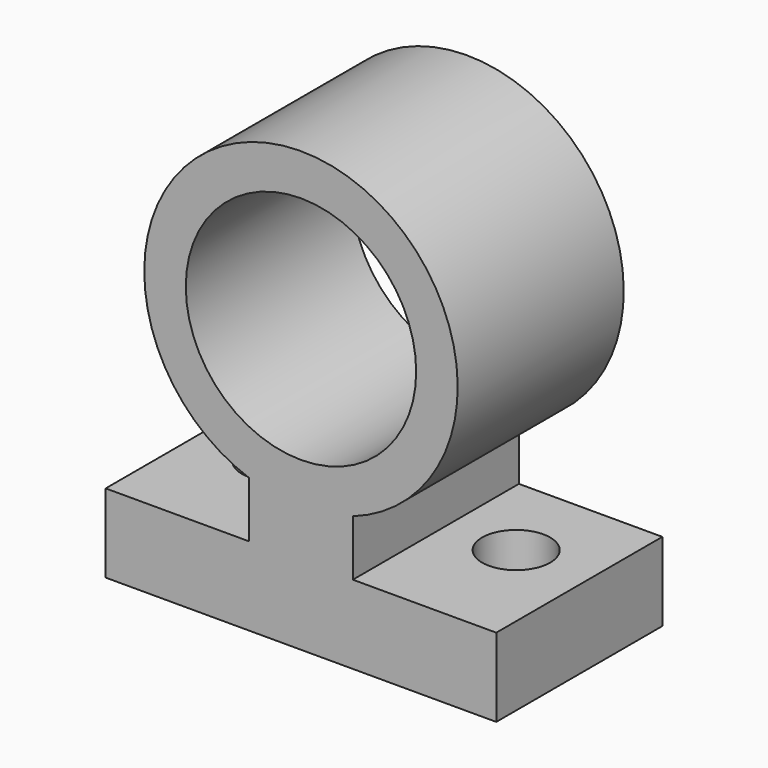
from build123d import *

# Parameters (mm, degrees)
F1_DEPTH = 25.4
F2_R     = 4.1683581246
F3_DEPTH = 10.668


# Not quite as in the source:
# - a feature names something its author has since deleted; it is built from what else it names


with BuildPart() as f1:
    # F0 (on Front) → F1 (new body)
    with BuildSketch(Plane.XZ):
        with BuildLine():
            ThreePointArc((6.35, -18.0951603751), (11.0901618338, 15.6449876798), (-19.177, 0))
            ThreePointArc((-19.177, 0), (-15.6449876798, -11.0901618338), (-6.35, -18.0951603751))
            Line((-6.35, -18.0951603751), (-6.35, -24.9301567674))
            Line((-6.35, -24.9301567674), (-23.899981752, -24.9301567674))
            Line((-23.899981752, -24.9301567674), (-23.899981752, -34.5450900495))
            Line((-23.899981752, -34.5450900495), (23.899981752, -34.5450900495))
            Line((23.899981752, -34.5450900495), (23.899981752, -24.9301567674))
            Line((23.899981752, -24.9301567674), (6.35, -24.9301567674))
            Line((6.35, -24.9301567674), (6.35, -18.0951603751))
        make_face()
        with BuildLine():
            ThreePointArc((-14.097, 0), (0, 14.097), (14.097, 0))
            ThreePointArc((14.097, 0), (0, -14.097), (-14.097, 0))
        make_face(mode=Mode.SUBTRACT)
    extrude(amount=F1_DEPTH)

    # F2 (on face) → F3 (cut)
    with BuildSketch(Plane(origin=(0, 0, -34.5450900495), x_dir=(1, 0, 0), z_dir=(0, 0, -1))):
        with Locations((-14.7024132311, 10.8604691923)):
            Circle(F2_R)
        with Locations((14.7024132311, 10.8604691923)):
            Circle(F2_R)
    extrude(amount=-F3_DEPTH, mode=Mode.SUBTRACT)


solid = f1.part
